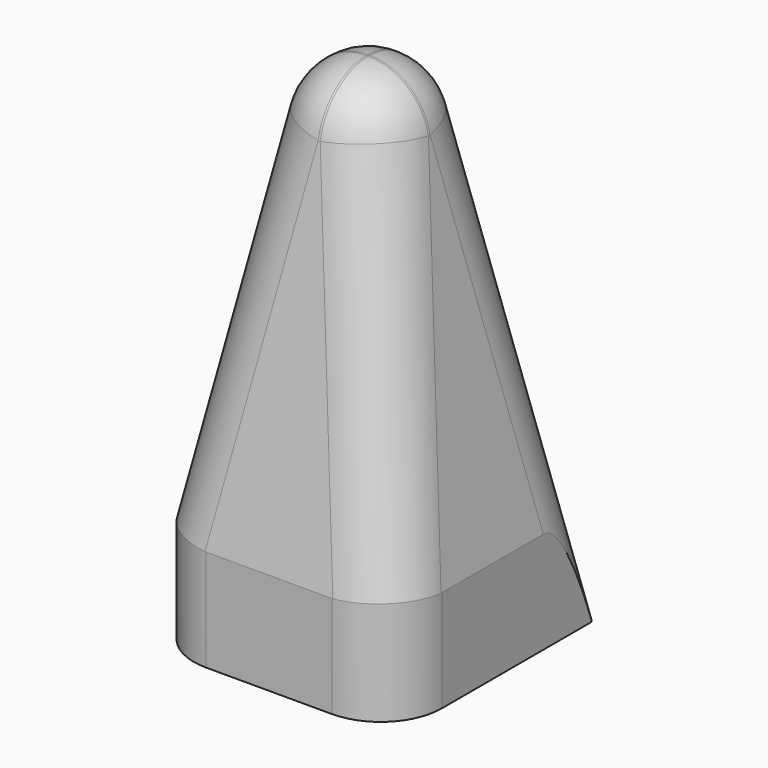
from build123d import *

# Parameters (mm, degrees)
F0_W         = 15.478125
F0_H         = 15.478125
F1_DEPTH     = 6.35
F2_DEPTH     = 25.4
F2_TAPER     = 10
F3_T1_DEPTH  = 51.3009034407
F3_T3_DEPTH  = 51.3009034407
F3_T5_DEPTH  = 51.3009034407
F3_T7_DEPTH  = 51.3009034407
F3_T9_DEPTH  = 44.45
F3_T11_DEPTH = 0.1267751904
F3_T13_DEPTH = 0.1267751904
F3_S17_W     = 14.1899336178
F3_S17_H     = 14.1899336178
F3_T18_DEPTH = 7.0949668089
F3_S29_W     = 14.1899336177
F3_S29_H     = 14.1899336178
F3_T30_DEPTH = 7.0949668089
F3_S41_W     = 14.1899336177
F3_S41_H     = 14.1899336178
F3_T42_DEPTH = 7.0949668089
F3_S53_W     = 14.1899336178
F3_S53_H     = 14.1899336178
F3_T54_DEPTH = 7.0949668089


# Not quite as in the source:
# - a fillet or chamfer that OpenCascade refuses, or shapes differently, is made with other operations: its cross-section is extruded or revolved along the edge and cut away or added


with BuildPart() as f1:
    # F0 (on Top) → F1 (new body)
    with BuildSketch(Plane.XY):
        with Locations((7.7390625, 7.7390625)):
            Rectangle(F0_W, F0_H)
    extrude(amount=-F1_DEPTH)

    # F0 (on Top) → F2 (join)
    with BuildSketch(Plane.XY):
        with Locations((7.7390625, 7.7390625)):
            Rectangle(F0_W, F0_H)
    extrude(amount=F2_DEPTH, taper=F2_TAPER)

    # F3: fillet of radius 3.81 on 10 edges, made by hand

    # F3_s2 → F3_t1 (cut)
    with BuildSketch(Plane(origin=(5.649698691, 5.649698691, -32.0410334724), x_dir=(0.7071067812, -0.7071067812, 0), z_dir=(-0.1710878697, -0.1710878697, 0.9702875252))):
        with BuildLine():
            ThreePointArc((-2.6531477556, 18.6646706441), (0, 19.7402772951), (2.6531477556, 18.6646706441))
            Line((2.6531477556, 18.6646706441), (0, 21.238986814))
            Line((0, 21.238986814), (-2.6531477556, 18.6646706441))
        make_face()
    extrude(amount=F3_T1_DEPTH, mode=Mode.SUBTRACT)

    # F3_s4 → F3_t3 (cut)
    with BuildSketch(Plane(origin=(-5.1966375782, 5.1966375782, -29.4715962203), x_dir=(0.7071067812, 0.7071067812, 0), z_dir=(0.1710878697, -0.1710878697, 0.9702875252))):
        with BuildLine():
            ThreePointArc((8.2915393919, 8.0451772371), (10.9446871476, 9.1207838881), (13.5978349032, 8.0451772371))
            Line((13.5978349032, 8.0451772371), (10.9446871476, 10.619493407))
            Line((10.9446871476, 10.619493407), (8.2915393919, 8.0451772371))
        make_face()
    extrude(amount=F3_T3_DEPTH, mode=Mode.SUBTRACT)

    # F3_s6 → F3_t5 (cut)
    with BuildSketch(Plane(origin=(5.1966375782, -5.1966375782, -29.4715962203), x_dir=(-0.7071067812, -0.7071067812, 0), z_dir=(-0.1710878697, 0.1710878697, 0.9702875252))):
        with BuildLine():
            ThreePointArc((-8.2915393919, 8.0451772371), (-10.9446871476, 9.1207838881), (-13.5978349032, 8.0451772371))
            Line((-13.5978349032, 8.0451772371), (-10.9446871476, 10.619493407))
            Line((-10.9446871476, 10.619493407), (-8.2915393919, 8.0451772371))
        make_face()
    extrude(amount=F3_T5_DEPTH, mode=Mode.SUBTRACT)

    # F3_s8 → F3_t7 (cut)
    with BuildSketch(Plane(origin=(-4.7435764654, -4.7435764654, -26.9021589682), x_dir=(-0.7071067812, 0.7071067812, 0), z_dir=(0.1710878697, 0.1710878697, 0.9702875252))):
        with BuildLine():
            ThreePointArc((2.6531477556, -2.5743161699), (0, -1.4987095189), (-2.6531477556, -2.5743161699))
            Line((-2.6531477556, -2.5743161699), (0, 0))
            Line((0, 0), (2.6531477556, -2.5743161699))
        make_face()
    extrude(amount=F3_T7_DEPTH, mode=Mode.SUBTRACT)

    # F3_s10 → F3_t9 (cut)
    with BuildSketch(Plane.XY.offset(-15.875)):
        with BuildLine():
            ThreePointArc((0, 3.81), (1.1159231637, 1.1159231637), (3.81, 0))
            Line((3.81, 0), (0, 0))
            Line((0, 0), (0, 3.81))
        make_face()
        with BuildLine():
            ThreePointArc((11.668125, 0), (14.3622018363, 1.1159231637), (15.478125, 3.81))
            Line((15.478125, 3.81), (15.478125, 0))
            Line((15.478125, 0), (11.668125, 0))
        make_face()
    extrude(amount=F3_T9_DEPTH, mode=Mode.SUBTRACT)

    # F3_s12 → F3_t11 (cut)
    with BuildSketch(Plane.XZ.offset(-7.8024500952)):
        with BuildLine():
            ThreePointArc((7.8024500952, 25.4), (10.2514708881, 24.5086293283), (11.5545676342, 22.2515995569))
            Line((11.5545676342, 22.2515995569), (10.99941969, 25.4))
            Line((10.99941969, 25.4), (7.8024500952, 25.4))
        make_face()
        with BuildLine():
            ThreePointArc((3.9235573658, 22.2515995569), (5.2266541119, 24.5086293283), (7.6756749048, 25.4))
            Line((7.6756749048, 25.4), (4.47870531, 25.4))
            Line((4.47870531, 25.4), (3.9235573658, 22.2515995569))
        make_face()
    extrude(amount=F3_T11_DEPTH, mode=Mode.SUBTRACT)

    # F3_s14 → F3_t13 (cut)
    with BuildSketch(Plane.YZ.offset(7.6756749048)):
        with BuildLine():
            ThreePointArc((3.9235573658, 22.2515995569), (5.2266541119, 24.5086293283), (7.6756749048, 25.4))
            Line((7.6756749048, 25.4), (4.47870531, 25.4))
            Line((4.47870531, 25.4), (3.9235573658, 22.2515995569))
        make_face()
        with BuildLine():
            ThreePointArc((11.5545676342, 22.2515995569), (10.2514708881, 24.5086293283), (7.8024500952, 25.4))
            Line((7.8024500952, 25.4), (10.99941969, 25.4))
            Line((10.99941969, 25.4), (11.5545676342, 22.2515995569))
        make_face()
    extrude(amount=F3_T13_DEPTH, mode=Mode.SUBTRACT)


with BuildPart() as f3_tool16:
    # F3_s17 → F3_t18 (new body)
    with BuildSketch(Plane(origin=(11.6595829736, 11.6595829736, 15.951248959), x_dir=(-0.7071067812, 0.7071067812, 0), z_dir=(0.5082206017, 0.5082206017, 0.6952867322))):
        with Locations((0, 7.8454102114)):
            Rectangle(F3_S17_W, F3_S17_H)
    extrude(amount=F3_T18_DEPTH)

    split(bisect_by=Plane.XZ.offset(-7.8024500952), keep=Keep.BOTTOM)

    split(bisect_by=Plane(origin=(-3.1272635948, -3.1272635948, 17.7355931701), x_dir=(0.7071067812, -0.7071067812, 0), z_dir=(-0.1710878697, -0.1710878697, 0.9702875252)), keep=Keep.TOP)

    split(bisect_by=Plane.YZ.offset(7.8024500952), keep=Keep.TOP)

    split(bisect_by=Plane.XY.offset(25.4), keep=Keep.BOTTOM)

    split(bisect_by=Plane(origin=(15.0114024231, 0, 2.6469152655), x_dir=(0, 1, 0), z_dir=(-0.984807753, 0, -0.1736481777)), keep=Keep.TOP)

    split(bisect_by=Plane(origin=(0, 15.0114024231, 2.6469152655), x_dir=(1, 0, 0), z_dir=(0, -0.984807753, -0.1736481777)), keep=Keep.TOP)

    # F3_s25 → F3_t26 (revolve, cut)
    with BuildSketch(Plane(origin=(7.8024500952, 7.8024500952, 21.59), x_dir=(-0.5082206017, -0.5082206017, -0.6952867322), z_dir=(-0.4916419632, -0.4916419632, 0.7187324676))):
        with BuildLine():
            ThreePointArc((0, -3.81), (3.81, 0), (0, 3.81))
            Line((0, 3.81), (0, -3.81))
        make_face()
    revolve(axis=Axis((7.8024500952, 7.8024500952, 21.59), (0.7071067812, -0.7071067812, 0)), mode=Mode.SUBTRACT)


with BuildPart() as f1_1:
    add(f1.part)

    # F3_t15: cut F3_tool16
    add(f3_tool16.part, mode=Mode.SUBTRACT)


with BuildPart() as f3_tool28:
    # F3_s29 → F3_t30 (new body)
    with BuildSketch(Plane(origin=(-7.6617662372, 7.6617662372, 10.4819135463), x_dir=(-0.7071067812, -0.7071067812, 0), z_dir=(-0.5082206017, 0.5082206017, 0.6952867322))):
        with Locations((-10.9446871475, 15.455105973)):
            Rectangle(F3_S29_W, F3_S29_H)
    extrude(amount=F3_T30_DEPTH)

    split(bisect_by=Plane.XZ.offset(-7.8024500952), keep=Keep.BOTTOM)

    split(bisect_by=Plane(origin=(3.5803247075, -3.5803247075, 20.3050304222), x_dir=(0.7071067812, 0.7071067812, 0), z_dir=(0.1710878697, -0.1710878697, 0.9702875252)), keep=Keep.TOP)

    split(bisect_by=Plane.YZ.offset(7.6756749048), keep=Keep.BOTTOM)

    split(bisect_by=Plane.XY.offset(25.4), keep=Keep.BOTTOM)

    split(bisect_by=Plane(origin=(0, 0, 0), x_dir=(0, 1, 0), z_dir=(0.984807753, 0, -0.1736481777)), keep=Keep.TOP)

    split(bisect_by=Plane(origin=(0, 15.0114024231, 2.6469152655), x_dir=(1, 0, 0), z_dir=(0, -0.984807753, -0.1736481777)), keep=Keep.TOP)

    # F3_s37 → F3_t38 (revolve, cut)
    with BuildSketch(Plane(origin=(7.6756749048, 7.8024500952, 21.59), x_dir=(0.5082206017, -0.5082206017, -0.6952867322), z_dir=(0.4916419632, -0.4916419632, 0.7187324676))):
        with BuildLine():
            ThreePointArc((0, -3.81), (3.81, 0), (0, 3.81))
            Line((0, 3.81), (0, -3.81))
        make_face()
    revolve(axis=Axis((7.6756749048, 7.8024500952, 21.59), (0.7071067812, 0.7071067812, 0)), mode=Mode.SUBTRACT)


with BuildPart() as f1_2:
    add(f1_1.part)

    # F3_t27: cut F3_tool28
    add(f3_tool28.part, mode=Mode.SUBTRACT)


with BuildPart() as f3_tool40:
    # F3_s41 → F3_t42 (new body)
    with BuildSketch(Plane(origin=(7.6617662372, -7.6617662372, 10.4819135463), x_dir=(0.7071067812, 0.7071067812, 0), z_dir=(0.5082206017, -0.5082206017, 0.6952867322))):
        with Locations((10.9446871475, 15.455105973)):
            Rectangle(F3_S41_W, F3_S41_H)
    extrude(amount=F3_T42_DEPTH)

    split(bisect_by=Plane.XZ.offset(-7.6756749048), keep=Keep.TOP)

    split(bisect_by=Plane(origin=(-3.5803247075, 3.5803247075, 20.3050304222), x_dir=(-0.7071067812, -0.7071067812, 0), z_dir=(-0.1710878697, 0.1710878697, 0.9702875252)), keep=Keep.TOP)

    split(bisect_by=Plane.YZ.offset(7.8024500952), keep=Keep.TOP)

    split(bisect_by=Plane.XY.offset(25.4), keep=Keep.BOTTOM)

    split(bisect_by=Plane(origin=(15.0114024231, 0, 2.6469152655), x_dir=(0, 1, 0), z_dir=(-0.984807753, 0, -0.1736481777)), keep=Keep.TOP)

    split(bisect_by=Plane(origin=(0, 0, 0), x_dir=(1, 0, 0), z_dir=(0, 0.984807753, -0.1736481777)), keep=Keep.TOP)

    # F3_s49 → F3_t50 (revolve, cut)
    with BuildSketch(Plane(origin=(7.8024500952, 7.6756749048, 21.59), x_dir=(-0.5082206017, 0.5082206017, -0.6952867322), z_dir=(-0.4916419632, 0.4916419632, 0.7187324676))):
        with BuildLine():
            ThreePointArc((0, -3.81), (3.81, 0), (0, 3.81))
            Line((0, 3.81), (0, -3.81))
        make_face()
    revolve(axis=Axis((7.8024500952, 7.6756749048, 21.59), (-0.7071067812, -0.7071067812, 0)), mode=Mode.SUBTRACT)


with BuildPart() as f1_3:
    add(f1_2.part)

    # F3_t39: cut F3_tool40
    add(f3_tool40.part, mode=Mode.SUBTRACT)


with BuildPart() as f3_tool52:
    # F3_s53 → F3_t54 (new body)
    with BuildSketch(Plane(origin=(-3.6639495007, -3.6639495007, 5.0125781335), x_dir=(0.7071067812, -0.7071067812, 0), z_dir=(-0.5082206017, -0.5082206017, 0.6952867322))):
        with Locations((0, 23.0648017346)):
            Rectangle(F3_S53_W, F3_S53_H)
    extrude(amount=F3_T54_DEPTH)

    split(bisect_by=Plane.XZ.offset(-7.6756749048), keep=Keep.TOP)

    split(bisect_by=Plane(origin=(4.0333858203, 4.0333858203, 22.8744676743), x_dir=(-0.7071067812, 0.7071067812, 0), z_dir=(0.1710878697, 0.1710878697, 0.9702875252)), keep=Keep.TOP)

    split(bisect_by=Plane.YZ.offset(7.6756749048), keep=Keep.BOTTOM)

    split(bisect_by=Plane.XY.offset(25.4), keep=Keep.BOTTOM)

    split(bisect_by=Plane(origin=(0, 0, 0), x_dir=(0, 1, 0), z_dir=(0.984807753, 0, -0.1736481777)), keep=Keep.TOP)

    split(bisect_by=Plane(origin=(0, 0, 0), x_dir=(1, 0, 0), z_dir=(0, 0.984807753, -0.1736481777)), keep=Keep.TOP)

    # F3_s61 → F3_t62 (revolve, cut)
    with BuildSketch(Plane(origin=(7.6756749048, 7.6756749048, 21.59), x_dir=(0.5082206017, 0.5082206017, -0.6952867322), z_dir=(0.4916419632, 0.4916419632, 0.7187324676))):
        with BuildLine():
            ThreePointArc((0, -3.81), (3.81, 0), (0, 3.81))
            Line((0, 3.81), (0, -3.81))
        make_face()
    revolve(axis=Axis((7.6756749048, 7.6756749048, 21.59), (-0.7071067812, 0.7071067812, 0)), mode=Mode.SUBTRACT)


with BuildPart() as f1_4:
    add(f1_3.part)

    # F3_t51: cut F3_tool52
    add(f3_tool52.part, mode=Mode.SUBTRACT)


solid = f1_4.part
